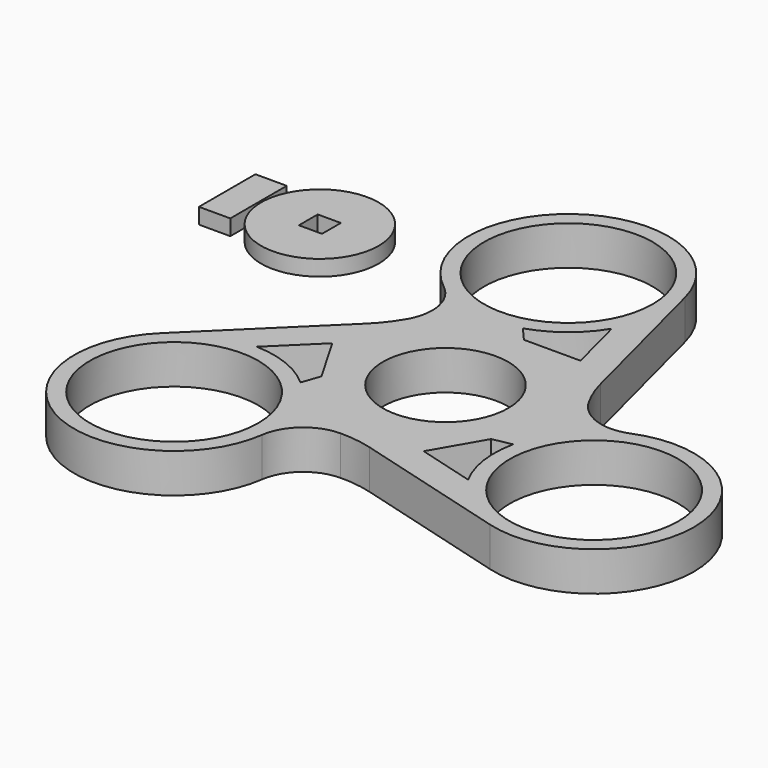
from build123d import *

# Parameters (mm, degrees)
F0_R        = 8
F1_DEPTH    = 5
F0_R_2      = 10.75
F2_DEPTH    = 5
F3_COUNT    = 3
F4_T1_DEPTH = 5
F5_W        = 4
F5_H        = 9
F6_DEPTH    = 2
F5_R        = 7.5
F5_W_2      = 2.95
F5_H_2      = 3
F7_R        = 6


# Not quite as in the source:
# - a fillet or chamfer that OpenCascade refuses, or shapes differently, is made with other operations: its cross-section is extruded or revolved along the edge and cut away or added
# - a feature names something its author has since deleted; it is built from what else it names


with BuildPart() as f1:
    # F0 (on Top) → F1 (new body)
    with BuildSketch(Plane.XY):
        Polygon((0, 12.5), (-7.2168783649, 12.5), (-14.4337567297, 0), (-7.2168783649, -12.5), (7.2168783649, -12.5), (14.4337567297, 0), (7.2168783649, 12.5), align=None)
        Circle(F0_R, mode=Mode.SUBTRACT)
    extrude(amount=F1_DEPTH)

    # F0 (on Top) → F2 (join)
    with BuildSketch(Plane.XY):
        with BuildLine():
            Line((-10.0093687347, 14.5615867092), (-7.2168783649, 12.5))
            Line((-7.2168783649, 12.5), (0, 12.5))
            Line((0, 12.5), (-1.6247319688, 14.3638148409))
            ThreePointArc((-1.6247319688, 14.3638148409), (2.3445854374, 16.4748201373), (5.3344467629, 19.8322824659))
            Line((5.3344467629, 19.8322824659), (7.2168783649, 12.5))
            Line((7.2168783649, 12.5), (14.4337567297, 0))
            Line((14.4337567297, 0), (6.8163861068, 29.6705139226))
            ThreePointArc((6.8163861068, 29.6705139226), (-14.0517470331, 35.9865969309), (-10.0093687347, 14.5615867092))
        make_face()
        with Locations((-5.5331216351, 26.5)):
            Circle(F0_R_2, mode=Mode.SUBTRACT)
    extrude(amount=F2_DEPTH)

    # F3: F1 ×3 about axis
    f3_axis = Axis((0, 0, 0), (0, 0, 1))


with BuildPart() as f1_1:
    add(f1.part)
    for i in range(1, F3_COUNT):
        add(f1.part.rotate(f3_axis, i * 360 / F3_COUNT))

    # F4: fillet of radius 15 on 3 edges, made by hand

    # F4_s2 → F4_t1 (join)
    with BuildSketch(Plane.XY):
        with BuildLine():
            ThreePointArc((2.5065087004, -15.21505791), (-2.6136621593, -14.7017722607), (-7.6060196422, -15.9491609547))
            Line((-7.6060196422, -15.9491609547), (-7.2168783649, -12.5))
            Line((-7.2168783649, -12.5), (2.5065087004, -15.21505791))
        make_face()
        with BuildLine():
            ThreePointArc((-14.4298810204, 5.4368287457), (-11.4252771788, 9.6143839572), (-10.0093687348, 14.5615867092))
            Line((-10.0093687348, 14.5615867092), (-7.2168783649, 12.5))
            Line((-7.2168783649, 12.5), (-14.4298810204, 5.4368287457))
        make_face()
        with BuildLine():
            ThreePointArc((11.92337232, 9.7782291644), (14.0389393381, 5.0873883035), (17.6153883769, 1.3875742456))
            Line((17.6153883769, 1.3875742456), (14.4337567297, 0))
            Line((14.4337567297, 0), (11.92337232, 9.7782291644))
        make_face()
    extrude(amount=F4_T1_DEPTH)

    # F7
    f7_edges = [f1_1.edges().sort_by_distance(p)[0] for p in [
        (-10.009369, 14.561587, 2.5),
        (17.615388, 1.387574, 2.5),
        (-7.60602, -15.949161, 2.5),
    ]]
    fillet(f7_edges, radius=F7_R)


with BuildPart() as f6:
    # F5 (on Top) → F6 (new body)
    with BuildSketch(Plane.XY):
        with Locations((-44.7917245328, 23.6781613976)):
            Rectangle(F5_W, F5_H)
    extrude(amount=F6_DEPTH)


with BuildPart() as f6b:
    # F5 (on Top) → F6, piece 2 (new body)
    with BuildSketch(Plane.XY):
        with Locations((-35.0555505693, 23.7860276699)):
            Circle(F5_R)
        with Locations((-35.0555505693, 23.7860276699)):
            Rectangle(F5_W_2, F5_H_2, mode=Mode.SUBTRACT)
    extrude(amount=F6_DEPTH)


solid = Compound([f1_1.part, f6.part, f6b.part])
